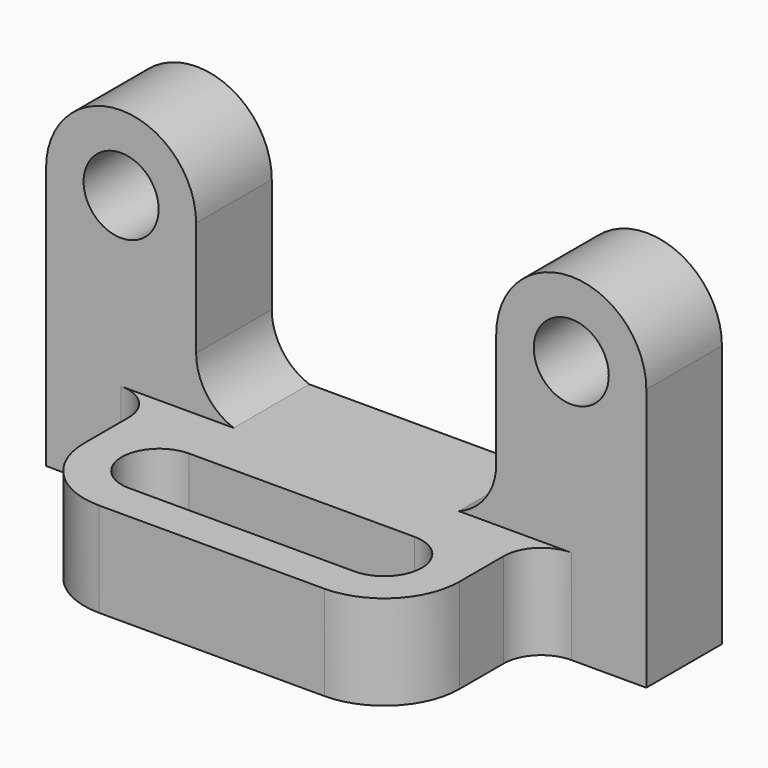
from build123d import *

# Parameters (mm, degrees)
F1_DEPTH = 16.002
F2_R     = 6.35
F3_DEPTH = 16.003
F6_DEPTH = 16.002
F4_W     = 38.1
F4_H     = 12.7
F7_DEPTH = 16.003


# Not quite as in the source:
# - a feature names something its author has since deleted; it is built from what else it names


with BuildPart() as f1:
    # F0 (on Front) → F1 (new body)
    with BuildSketch(Plane.XZ):
        with BuildLine():
            Line((0, 44.45), (0, 0))
            Line((0, 0), (101.6, 0))
            Line((101.6, 0), (101.6, 44.45))
            Line((101.6, 44.45), (76.2, 44.45))
            Line((76.2, 44.45), (76.2, 25.0716141042))
            ThreePointArc((76.2, 25.0716141042), (74.4547062675, 19.535812446), (69.85, 16.002))
            Line((69.85, 16.002), (31.75, 16.002))
            ThreePointArc((31.75, 16.002), (27.1452937325, 19.535812446), (25.4, 25.0716141042))
            Line((25.4, 25.0716141042), (25.4, 44.45))
            Line((25.4, 44.45), (0, 44.45))
        make_face()
        with BuildLine():
            ThreePointArc((25.4, 44.45), (12.7, 57.15), (0, 44.45))
            Line((0, 44.45), (25.4, 44.45))
        make_face()
        with BuildLine():
            Line((76.2, 44.45), (101.6, 44.45))
            ThreePointArc((101.6, 44.45), (88.9, 57.15), (76.2, 44.45))
        make_face()
    extrude(amount=F1_DEPTH)

    # F2 (on face) → F3 (cut, through all)
    with BuildSketch(Plane.XZ.offset(16.002)):
        with Locations((12.7, 44.45)):
            Circle(F2_R)
        with Locations((88.9, 44.45)):
            Circle(F2_R)
    extrude(amount=-F3_DEPTH, mode=Mode.SUBTRACT)

    # F5 (on Top) → F6 (join)
    with BuildSketch(Plane.XY):
        with BuildLine():
            ThreePointArc((19.05, -31.75), (22.7697438789, -40.7302561211), (31.75, -44.45))
            Line((31.75, -44.45), (69.85, -44.45))
            ThreePointArc((69.85, -44.45), (78.8302561211, -40.7302561211), (82.55, -31.75))
            Line((82.55, -31.75), (82.55, -22.352))
            Line((82.55, -22.352), (82.55, -16.002))
            Line((82.55, -16.002), (19.05, -16.002))
            Line((19.05, -16.002), (19.05, -22.352))
            Line((19.05, -22.352), (19.05, -31.75))
        make_face()
        with BuildLine():
            ThreePointArc((12.7, -16.002), (17.1901280605, -17.8618719395), (19.05, -22.352))
            Line((19.05, -22.352), (19.05, -16.002))
            Line((19.05, -16.002), (12.7, -16.002))
        make_face()
        with BuildLine():
            Line((82.55, -16.002), (82.55, -22.352))
            ThreePointArc((82.55, -22.352), (84.4098719395, -17.8618719395), (88.9, -16.002))
            Line((88.9, -16.002), (82.55, -16.002))
        make_face()
    extrude(amount=F6_DEPTH)

    # F4 (on face) → F7 (cut, through all)
    with BuildSketch(Plane.XY.offset(16.002)):
        with Locations((50.8, -31.75)):
            Rectangle(F4_W, F4_H)
        with BuildLine():
            Line((31.75, -38.1), (31.75, -25.4))
            ThreePointArc((31.75, -25.4), (25.4, -31.75), (31.75, -38.1))
        make_face()
        with BuildLine():
            ThreePointArc((69.85, -38.1), (76.2, -31.75), (69.85, -25.4))
            Line((69.85, -25.4), (69.85, -38.1))
        make_face()
    extrude(amount=-F7_DEPTH, mode=Mode.SUBTRACT)


solid = f1.part
